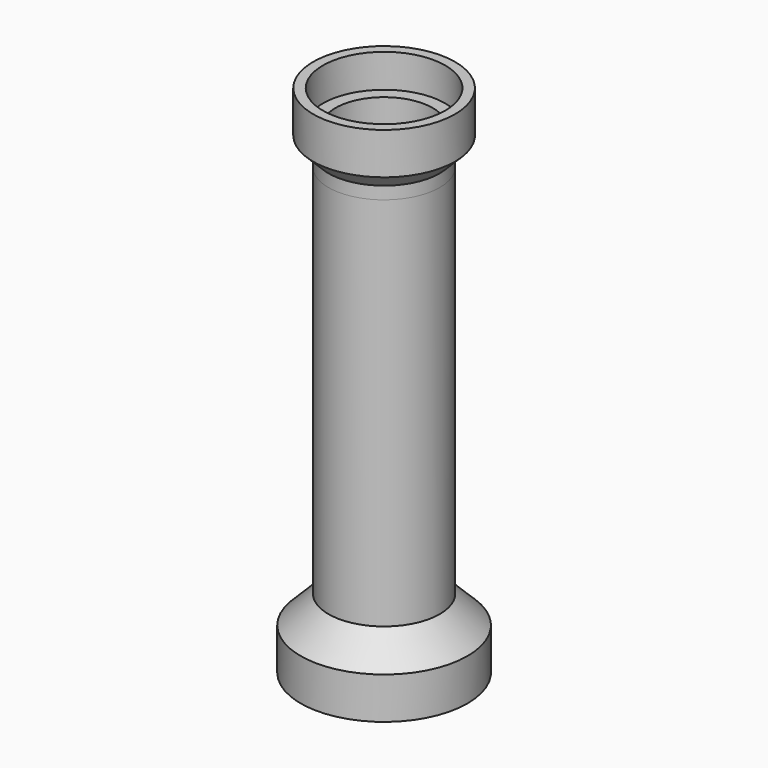
from build123d import *

# Parameters (mm, degrees)
F0_R          = 20
F0_R_2        = 17.5
F1_DEPTH      = 135
F2_R          = 30
F2_R_2        = 26.9985
F2_R_3        = 17.5
F3_DEPTH      = 25
F4_R          = 26.9965
F4_R_2        = 24
F4_R_3        = 17.5
F5_DEPTH      = 12
F6_R          = 25.5
F6_R_2        = 22.4965
F6_R_3        = 20
F6_R_4        = 17.5
F7_DEPTH      = 25
F8_R          = 21.9965
F8_R_2        = 17.5
F9_DEPTH      = 12
F10_S5_R      = 20
F10_T6_DEPTH  = 38
F10_S11_R     = 20
F10_T12_DEPTH = 44


# Not quite as in the source:
# - a fillet or chamfer that OpenCascade refuses, or shapes differently, is made with other operations: its cross-section is extruded or revolved along the edge and cut away or added


with BuildPart() as f1:
    # F0 (on Top) → F1 (new body)
    with BuildSketch(Plane.XY):
        Circle(F0_R)
        Circle(F0_R_2, mode=Mode.SUBTRACT)
    extrude(amount=F1_DEPTH)

    # F2 (on Top) → F3 (join)
    with BuildSketch(Plane.XY):
        Circle(F2_R)
        Circle(F2_R_2, mode=Mode.SUBTRACT)
        Circle(F2_R_2)
        Circle(F2_R_3, mode=Mode.SUBTRACT)
    extrude(amount=-F3_DEPTH)

    # F4 (on face) → F5 (cut)
    with BuildSketch(Plane(origin=(0, 0, -25), x_dir=(1, 0, 0), z_dir=(0, 0, -1))):
        Circle(F4_R)
        Circle(F4_R_2, mode=Mode.SUBTRACT)
        Circle(F4_R_2)
        Circle(F4_R_3, mode=Mode.SUBTRACT)
    extrude(amount=-F5_DEPTH, mode=Mode.SUBTRACT)

    # F6 (on face) → F7 (join)
    with BuildSketch(Plane.XY.offset(135)):
        Circle(F6_R)
        Circle(F6_R_2, mode=Mode.SUBTRACT)
        Circle(F6_R_2)
        Circle(F6_R_3, mode=Mode.SUBTRACT)
        Circle(F6_R_3)
        Circle(F6_R_4, mode=Mode.SUBTRACT)
    extrude(amount=F7_DEPTH)

    # F8 (on face) → F9 (cut)
    with BuildSketch(Plane.XY.offset(160)):
        Circle(F8_R)
        Circle(F8_R_2, mode=Mode.SUBTRACT)
    extrude(amount=-F9_DEPTH, mode=Mode.SUBTRACT)

    # F10: chamfer of 10 on 2 edges, made by hand


with BuildPart() as f10_tool2:
    # F10_s3 → F10_t4 (revolve)
    with BuildSketch(Plane.XZ):
        Polygon((15.5, 135), (25.5, 145), (25.5, 135), align=None)
    revolve(axis=Axis((0, 0, 135), (0, 0, 1)))

    # F10_s5 → F10_t6 (cut, symmetric)
    with BuildSketch(Plane.XY.offset(140)):
        Circle(F10_S5_R)
    extrude(amount=F10_T6_DEPTH, both=True, mode=Mode.SUBTRACT)


with BuildPart() as f1_1:
    add(f1.part)

    # F10_t1: cut F10_tool2
    add(f10_tool2.part, mode=Mode.SUBTRACT)


with BuildPart() as f10_tool8:
    # F10_s9 → F10_t10 (revolve)
    with BuildSketch(Plane.XZ):
        Polygon((20, 0), (30, -10), (30, 0), align=None)
    revolve(axis=Axis((0, 0, 0), (0, 0, 1)))

    # F10_s11 → F10_t12 (cut, symmetric)
    with BuildSketch(Plane.XY.offset(-5)):
        Circle(F10_S11_R)
    extrude(amount=F10_T12_DEPTH, both=True, mode=Mode.SUBTRACT)


with BuildPart() as f1_2:
    add(f1_1.part)

    # F10_t7: cut F10_tool8
    add(f10_tool8.part, mode=Mode.SUBTRACT)


solid = f1_2.part
